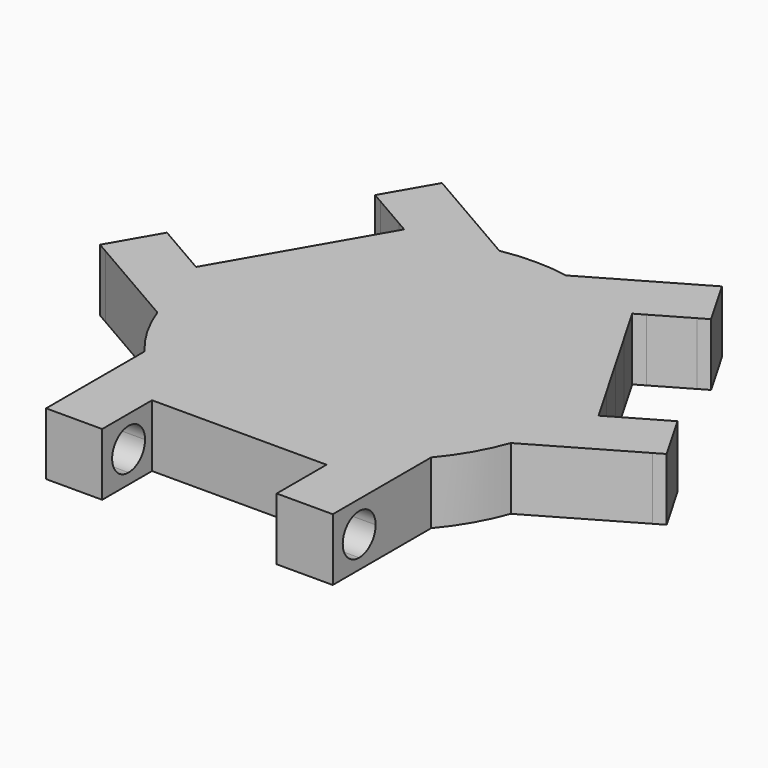
from build123d import *

# Parameters (mm, degrees)
F0_W     = 9
F0_H     = 6.4
F0_H_2   = 1.8
F1_DEPTH = 10
F3_DEPTH = 68.4572498646


with BuildPart() as f1:
    # F0 (on Top) → F1 (new body)
    with BuildSketch(Plane.XY):
        with BuildLine():
            Line((-23, -13.2790561914), (-23, -19.4471))
            Line((-23, -19.4471), (-23, -19.4592028655))
            ThreePointArc((-23, -19.4592028655), (-15.9535433508, -25.5567022661), (-7.3808786516, -29.2093))
            Line((-7.3808786516, -29.2093), (0, -29.2093))
            Line((0, -29.2093), (0, 0))
            Line((0, 0), (-11.5, -19.918584287))
            Line((-11.5, -19.918584287), (-23, -13.2790561914))
        make_face()
        with BuildLine():
            Line((-23, -19.4592028655), (-23, -19.4471))
            Line((-23, -19.4471), (-23, -13.2790561914))
            Line((-23, -13.2790561914), (-28.3416826299, -10.195034287))
            Line((-28.3416826299, -10.195034287), (-28.3521640189, -10.1889828543))
            ThreePointArc((-28.3521640189, -10.1889828543), (-26.0910987143, -15.0637028662), (-23, -19.4592028655))
        make_face()
        with BuildLine():
            ThreePointArc((-7.3808786516, -29.2093), (-15.9535433508, -25.5567022661), (-23, -19.4592028655))
            Line((-23, -19.4592028655), (-23, -31.0093))
            Line((-23, -31.0093), (-14, -31.0093))
            Line((-14, -31.0093), (-14, -29.2093))
            Line((-14, -29.2093), (-7.3808786516, -29.2093))
        make_face()
        with BuildLine():
            Line((-28.3416826299, -10.195034287), (-23, -13.2790561914))
            Line((-23, -13.2790561914), (-23, 0))
            Line((-23, 0), (0, 0))
            Line((0, 0), (-25.2959958268, 14.60465))
            Line((-25.2959958268, 14.60465), (-28.9864351526, 8.2126215854))
            ThreePointArc((-28.9864351526, 8.2126215854), (-30.1095250747, -1.0378226891), (-28.3521640189, -10.1889828543))
            Line((-28.3521640189, -10.1889828543), (-28.3416826299, -10.195034287))
        make_face()
        Polygon((-23, 0), (-23, -13.2790561914), (-11.5, -19.918584287), (0, 0), align=None)
        with Locations((-18.5, -34.2093)):
            Rectangle(F0_W, F0_H)
        with BuildLine():
            Line((-38.3548415536, -4.413934287), (-28.3521640189, -10.1889828543))
            ThreePointArc((-28.3521640189, -10.1889828543), (-30.1095250747, -1.0378226891), (-28.9864351526, 8.2126215854))
            Line((-28.9864351526, 8.2126215854), (-32.2959958268, 2.480294347))
            Line((-32.2959958268, 2.480294347), (-33.8548415536, 3.380294347))
            Line((-33.8548415536, 3.380294347), (-38.3548415536, -4.413934287))
        make_face()
        with Locations((-18.5, -38.3093)):
            Rectangle(F0_W, F0_H_2)
        Polygon((-43.8974041378, -1.213934287), (-38.3548415536, -4.413934287), (-33.8548415536, 3.380294347), (-39.3974041378, 6.580294347), align=None)
        with BuildLine():
            Line((0, 0), (0, -29.2093))
            Line((0, -29.2093), (7.3808786516, -29.2093))
            ThreePointArc((7.3808786516, -29.2093), (15.9535433508, -25.5567022661), (23, -19.4592028655))
            Line((23, -19.4592028655), (23, -19.4471))
            Line((23, -19.4471), (23, -13.2790561914))
            Line((23, -13.2790561914), (11.5, -19.918584287))
            Line((11.5, -19.918584287), (0, 0))
        make_face()
        with BuildLine():
            Line((25.2959958268, 14.60465), (0, 0))
            Line((0, 0), (23, 0))
            Line((23, 0), (23, -13.2790561914))
            Line((23, -13.2790561914), (28.3416826299, -10.195034287))
            Line((28.3416826299, -10.195034287), (28.3521640189, -10.1889828543))
            ThreePointArc((28.3521640189, -10.1889828543), (29.6802773315, -5.1712390862), (30.1274057323, 0))
            ThreePointArc((30.1274057323, 0), (29.8407998279, 4.1457498468), (28.9864351526, 8.2126215854))
            Line((28.9864351526, 8.2126215854), (25.2959958268, 14.60465))
        make_face()
        with BuildLine():
            Line((11.5, 19.918584287), (0, 0))
            Line((0, 0), (25.2959958268, 14.60465))
            Line((25.2959958268, 14.60465), (21.6055565009, 20.9966784146))
            ThreePointArc((21.6055565009, 20.9966784146), (14.155981724, 26.5945249552), (5.3521640189, 29.6481857198))
            Line((5.3521640189, 29.6481857198), (5.3416826299, 29.642134287))
            Line((5.3416826299, 29.642134287), (0, 26.5581123827))
            Line((0, 26.5581123827), (11.5, 19.918584287))
        make_face()
        with BuildLine():
            Line((-25.2959958268, 14.60465), (0, 0))
            Line((0, 0), (-11.5, 19.918584287))
            Line((-11.5, 19.918584287), (0, 26.5581123827))
            Line((0, 26.5581123827), (-5.3416826299, 29.642134287))
            Line((-5.3416826299, 29.642134287), (-5.3521640189, 29.6481857198))
            ThreePointArc((-5.3521640189, 29.6481857198), (-14.155981724, 26.5945249552), (-21.6055565009, 20.9966784146))
            Line((-21.6055565009, 20.9966784146), (-25.2959958268, 14.60465))
        make_face()
        Polygon((23, 0), (0, 0), (11.5, -19.918584287), (23, -13.2790561914), align=None)
        Polygon((-11.5, 19.918584287), (0, 0), (11.5, 19.918584287), (0, 26.5581123827), align=None)
        Polygon((-45.4562498646, -0.313934287), (-43.8974041378, -1.213934287), (-39.3974041378, 6.580294347), (-40.9562498646, 7.480294347), align=None)
        with BuildLine():
            ThreePointArc((23, -19.4592028655), (15.9535433508, -25.5567022661), (7.3808786516, -29.2093))
            Line((7.3808786516, -29.2093), (14, -29.2093))
            Line((14, -29.2093), (14, -31.0093))
            Line((14, -31.0093), (23, -31.0093))
            Line((23, -31.0093), (23, -19.4592028655))
        make_face()
        with Locations((18.5, -34.2093)):
            Rectangle(F0_W, F0_H)
        with BuildLine():
            Line((-18.2959958268, 26.729005653), (-21.6055565009, 20.9966784146))
            ThreePointArc((-21.6055565009, 20.9966784146), (-14.155981724, 26.5945249552), (-5.3521640189, 29.6481857198))
            Line((-5.3521640189, 29.6481857198), (-15.3548415536, 35.423234287))
            Line((-15.3548415536, 35.423234287), (-19.8548415536, 27.629005653))
            Line((-19.8548415536, 27.629005653), (-18.2959958268, 26.729005653))
        make_face()
        with BuildLine():
            Line((23, -19.4471), (23, -19.4592028655))
            ThreePointArc((23, -19.4592028655), (26.0910987143, -15.0637028662), (28.3521640189, -10.1889828543))
            Line((28.3521640189, -10.1889828543), (28.3416826299, -10.195034287))
            Line((28.3416826299, -10.195034287), (23, -13.2790561914))
            Line((23, -13.2790561914), (23, -19.4471))
        make_face()
        with BuildLine():
            ThreePointArc((5.3521640189, 29.6481857198), (14.155981724, 26.5945249552), (21.6055565009, 20.9966784146))
            Line((21.6055565009, 20.9966784146), (18.2959958268, 26.729005653))
            Line((18.2959958268, 26.729005653), (19.8548415536, 27.629005653))
            Line((19.8548415536, 27.629005653), (15.3548415536, 35.423234287))
            Line((15.3548415536, 35.423234287), (5.3521640189, 29.6481857198))
        make_face()
        with BuildLine():
            Line((32.2959958268, 2.480294347), (28.9864351526, 8.2126215854))
            ThreePointArc((28.9864351526, 8.2126215854), (29.8407998279, 4.1457498468), (30.1274057323, 0))
            ThreePointArc((30.1274057323, 0), (29.6802773315, -5.1712390862), (28.3521640189, -10.1889828543))
            Line((28.3521640189, -10.1889828543), (38.3548415536, -4.413934287))
            Line((38.3548415536, -4.413934287), (33.8548415536, 3.380294347))
            Line((33.8548415536, 3.380294347), (32.2959958268, 2.480294347))
        make_face()
        with BuildLine():
            Line((-5.3416826299, 29.642134287), (0, 26.5581123827))
            Line((0, 26.5581123827), (5.3416826299, 29.642134287))
            Line((5.3416826299, 29.642134287), (5.3521640189, 29.6481857198))
            ThreePointArc((5.3521640189, 29.6481857198), (0, 30.1274057323), (-5.3521640189, 29.6481857198))
            Line((-5.3521640189, 29.6481857198), (-5.3416826299, 29.642134287))
        make_face()
        with Locations((18.5, -38.3093)):
            Rectangle(F0_W, F0_H_2)
        Polygon((-25.3974041378, 30.829005653), (-19.8548415536, 27.629005653), (-15.3548415536, 35.423234287), (-20.8974041378, 38.623234287), align=None)
        Polygon((-26.9562498646, 31.729005653), (-25.3974041378, 30.829005653), (-20.8974041378, 38.623234287), (-22.4562498646, 39.523234287), align=None)
        Polygon((33.8548415536, 3.380294347), (38.3548415536, -4.413934287), (43.8974041378, -1.213934287), (39.3974041378, 6.580294347), align=None)
        Polygon((15.3548415536, 35.423234287), (19.8548415536, 27.629005653), (25.3974041378, 30.829005653), (20.8974041378, 38.623234287), align=None)
        Polygon((39.3974041378, 6.580294347), (43.8974041378, -1.213934287), (45.4562498646, -0.313934287), (40.9562498646, 7.480294347), align=None)
        Polygon((20.8974041378, 38.623234287), (25.3974041378, 30.829005653), (26.9562498646, 31.729005653), (22.4562498646, 39.523234287), align=None)
    extrude(amount=-F1_DEPTH)

    # F2 (on face) → F3 (cut, through all)
    with BuildSketch(Plane.YZ.offset(23)):
        with BuildLine():
            ThreePointArc((-33.9093, -1.7), (-37.2093, -5), (-33.9093, -8.3))
            Line((-33.9093, -8.3), (-33.9093, -1.7))
        make_face()
        with BuildLine():
            Line((-33.9093, -1.7), (-33.9093, -8.3))
            ThreePointArc((-33.9093, -8.3), (-31.5758476221, -7.3334523779), (-30.6093, -5))
            ThreePointArc((-30.6093, -5), (-31.5758476221, -2.6665476221), (-33.9093, -1.7))
        make_face()
    extrude(amount=-F3_DEPTH, mode=Mode.SUBTRACT)


solid = f1.part
